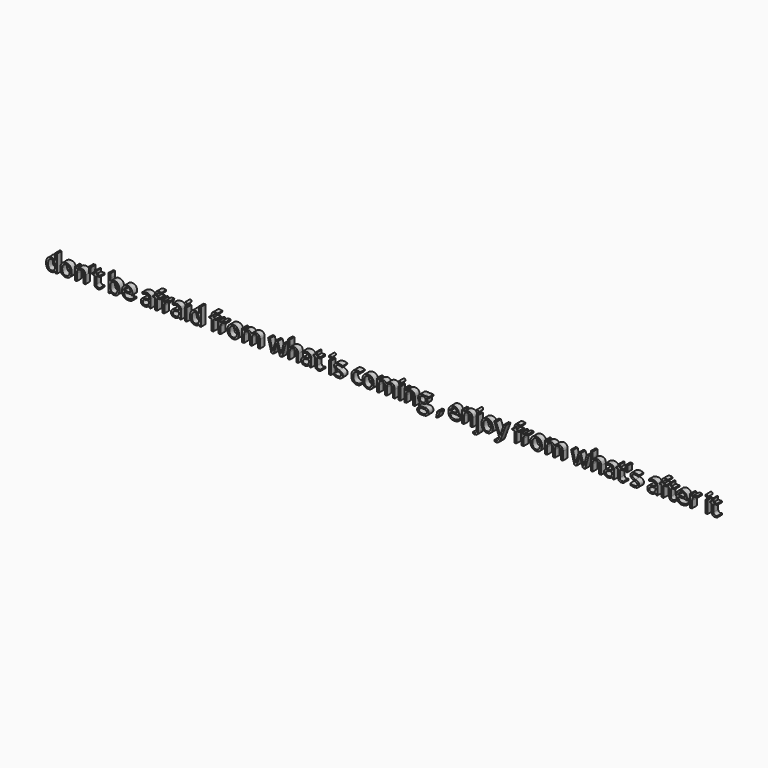
from build123d import *

# Parameters (mm, degrees)
F0_TEXT_SIZE = 98.2034899708
F1_DEPTH     = 25


# Not quite as in the source:
# - Text() gives the source's letters only with a copy of the font that has no kerning and outlines rounded to 1/6400 em; it was checked with that copy


with BuildPart() as f1:
    # F0 (on Front) → F1 (new body)
    with BuildSketch(Plane.XZ):
        with Locations((-82.8500166535, -30.8484081179)):
            Text("don't be afraid from what is coming , enjoy from what's after it", F0_TEXT_SIZE, font='Open Sans', text_align=(TextAlign.LEFT, TextAlign.BOTTOM))
    extrude(amount=F1_DEPTH)


solid = f1.part
